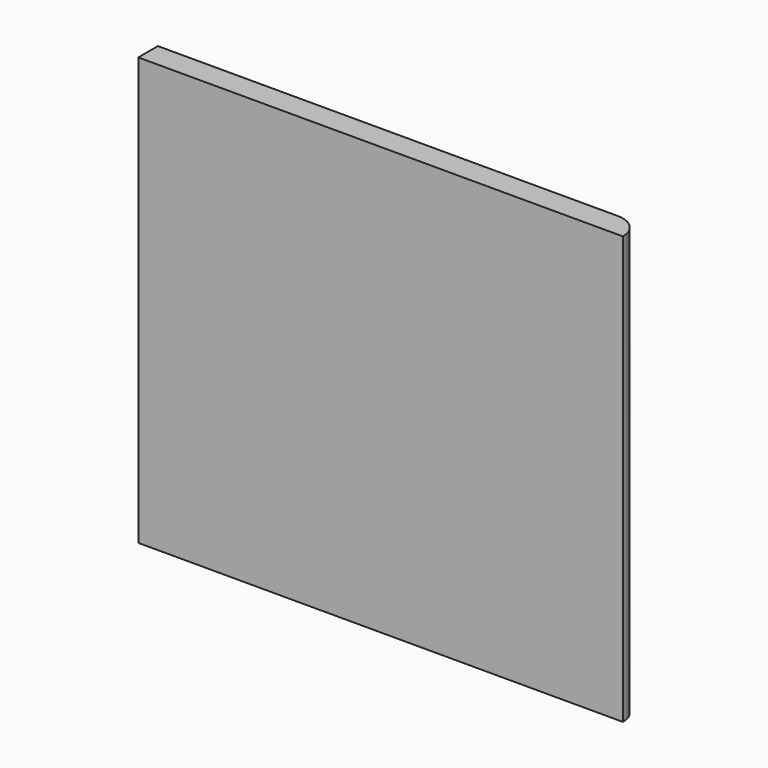
from build123d import *

# Parameters (mm, degrees)
F0_W     = 356
F0_H     = 314
F1_DEPTH = 18
F3_DEPTH = 5
F4_R     = 17.99999


# Not quite as in the source:
# - a fillet or chamfer is up to 0.001 mm smaller than in the source, because OpenCascade refuses the exact size


with BuildPart() as f1:
    # F0 (on Front) → F1 (new body)
    with BuildSketch(Plane.XZ):
        Rectangle(F0_W, F0_H)
    extrude(amount=F1_DEPTH)

    # F2 (on face) → F3 (cut)
    with BuildSketch(Plane(origin=(0, 0, 0), x_dir=(-1, 0, 0), z_dir=(0, 1, 0))):
        with BuildLine():
            ThreePointArc((28.5, -9), (37.5, 0), (28.5, 9))
            Line((28.5, 9), (-28.5, 9))
            ThreePointArc((-28.5, 9), (-37.5, 0), (-28.5, -9))
            Line((-28.5, -9), (28.5, -9))
        make_face()
    extrude(amount=-F3_DEPTH, mode=Mode.SUBTRACT)

    # F4 (radius 18 in the source; OpenCascade refuses exactly that, so slightly less here)
    f4_edges = [f1.edges().sort_by_distance(p)[0] for p in [
        (178, 0, 0),
    ]]
    fillet(f4_edges, radius=F4_R)


solid = f1.part
